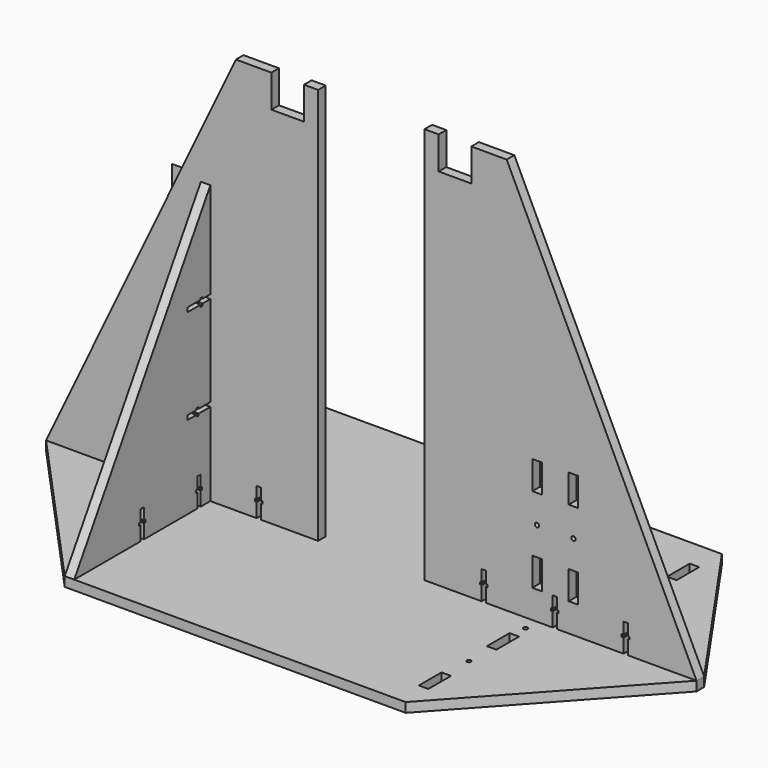
from build123d import *

# Parameters (mm, degrees)
F0_W     = 6.7
F0_H     = 20
F0_R     = 1.5
F1_DEPTH = 6.7
F3_DEPTH = 6.7
F4_R     = 1.5
F5_DEPTH = 25
F7_DEPTH = 6.7
F8_W     = 6.7
F8_H     = 20
F8_R     = 1.5
F8_W_2   = 20
F8_H_2   = 6.7
F9_DEPTH = 6.7


with BuildPart() as f1:
    # F0 (on Front) → F1 (new body)
    with BuildSketch(Plane.XZ):
        Polygon((-55.1449356675, 306.105045557), (-65.1449356675, 306.105045557), (-65.1449356675, 283.105045557), (-88.1449356675, 283.105045557), (-88.1449356675, 306.105045557), (-113.1449356675, 306.105045557), (-247.0069974661, 26.105045557), (-222.0069974661, 26.105045557), (-222.0069974661, 19.405045557), (-202.0069974661, 19.405045557), (-202.0069974661, 26.105045557), (-198.5069974661, 26.105045557), (-198.5069974661, 36.105045557), (-199.7569974661, 36.105045557), (-199.7569974661, 37.905045557), (-198.5069974661, 37.905045557), (-198.5069974661, 46.105045557), (-195.5069974661, 46.105045557), (-195.5069974661, 37.905045557), (-194.2569974661, 37.905045557), (-194.2569974661, 36.105045557), (-195.5069974661, 36.105045557), (-195.5069974661, 26.105045557), (-192.0069974661, 26.105045557), (-192.0069974661, 19.405045557), (-172.0069974661, 19.405045557), (-172.0069974661, 26.105045557), (-148.5069974661, 26.105045557), (-148.5069974661, 36.105045557), (-149.7569974661, 36.105045557), (-149.7569974661, 37.905045557), (-148.5069974661, 37.905045557), (-148.5069974661, 46.105045557), (-145.5069974661, 46.105045557), (-145.5069974661, 37.905045557), (-144.2569974661, 37.905045557), (-144.2569974661, 36.105045557), (-145.5069974661, 36.105045557), (-145.5069974661, 26.105045557), (-122.0069974661, 26.105045557), (-122.0069974661, 19.405045557), (-102.0069974661, 19.405045557), (-102.0069974661, 26.105045557), (-98.5069974661, 26.105045557), (-98.5069974661, 36.105045557), (-99.7569974661, 36.105045557), (-99.7569974661, 37.905045557), (-98.5069974661, 37.905045557), (-98.5069974661, 46.105045557), (-95.5069974661, 46.105045557), (-95.5069974661, 37.905045557), (-94.2569974661, 37.905045557), (-94.2569974661, 36.105045557), (-95.5069974661, 36.105045557), (-95.5069974661, 26.105045557), (-92.0069974661, 26.105045557), (-92.0069974661, 19.405045557), (-72.0069974661, 19.405045557), (-72.0069974661, 26.105045557), (-55.1449356675, 26.105045557), align=None)
        with Locations((-160.2069974661, 56.105045557)):
            Rectangle(F0_W, F0_H, mode=Mode.SUBTRACT)
        with Locations((-134.5069974661, 56.105045557)):
            Rectangle(F0_W, F0_H, mode=Mode.SUBTRACT)
        with Locations((-160.2069974661, 86.105045557)):
            Circle(F0_R, mode=Mode.SUBTRACT)
        with Locations((-134.5069974661, 86.105045557)):
            Circle(F0_R, mode=Mode.SUBTRACT)
        with Locations((-160.2069974661, 116.105045557)):
            Rectangle(F0_W, F0_H, mode=Mode.SUBTRACT)
        with Locations((-134.5069974661, 116.105045557)):
            Rectangle(F0_W, F0_H, mode=Mode.SUBTRACT)
    extrude(amount=F1_DEPTH)

    # F4 (on face) → F5 (cut)
    with BuildSketch(Plane(origin=(0, 0, 0), x_dir=(-1, 0, 0), z_dir=(0, 1, 0))):
        with Locations((134.5069974661, 153.039291501)):
            Circle(F4_R)
        with Locations((160.2069974661, 153.039291501)):
            Circle(F4_R)
        with Locations((-99.2171261311, 153.039291501)):
            Circle(F4_R)
        with Locations((-124.9171261311, 153.039291501)):
            Circle(F4_R)
    extrude(amount=-F5_DEPTH, mode=Mode.SUBTRACT)


with BuildPart() as f1b:
    # F0 (on Front) → F1, piece 2 (new body)
    with BuildSketch(Plane.XZ):
        Polygon((158.9671261311, 36.105045557), (158.9671261311, 37.905045557), (160.2171261311, 37.905045557), (160.2171261311, 46.105045557), (163.2171261311, 46.105045557), (163.2171261311, 37.905045557), (164.4671261311, 37.905045557), (164.4671261311, 36.105045557), (163.2171261311, 36.105045557), (163.2171261311, 26.105045557), (166.7171261311, 26.105045557), (166.7171261311, 19.405045557), (186.7171261311, 19.405045557), (186.7171261311, 26.105045557), (211.7171261311, 26.105045557), (77.8550643325, 306.105045557), (52.8550643325, 306.105045557), (52.8550643325, 283.105045557), (29.8550643325, 283.105045557), (29.8550643325, 306.105045557), (19.8550643325, 306.105045557), (19.8550643325, 26.105045557), (36.7171261311, 26.105045557), (36.7171261311, 19.405045557), (56.7171261311, 19.405045557), (56.7171261311, 26.105045557), (60.2171261311, 26.105045557), (60.2171261311, 36.105045557), (58.9671261311, 36.105045557), (58.9671261311, 37.905045557), (60.2171261311, 37.905045557), (60.2171261311, 46.105045557), (63.2171261311, 46.105045557), (63.2171261311, 37.905045557), (64.4671261311, 37.905045557), (64.4671261311, 36.105045557), (63.2171261311, 36.105045557), (63.2171261311, 26.105045557), (66.7171261311, 26.105045557), (66.7171261311, 19.405045557), (86.7171261311, 19.405045557), (86.7171261311, 26.105045557), (110.2171261311, 26.105045557), (110.2171261311, 36.105045557), (108.9671261311, 36.105045557), (108.9671261311, 37.905045557), (110.2171261311, 37.905045557), (110.2171261311, 46.105045557), (113.2171261311, 46.105045557), (113.2171261311, 37.905045557), (114.4671261311, 37.905045557), (114.4671261311, 36.105045557), (113.2171261311, 36.105045557), (113.2171261311, 26.105045557), (136.7171261311, 26.105045557), (136.7171261311, 19.405045557), (156.7171261311, 19.405045557), (156.7171261311, 26.105045557), (160.2171261311, 26.105045557), (160.2171261311, 36.105045557), align=None)
        with Locations((99.2171261311, 56.105045557)):
            Rectangle(F0_W, F0_H, mode=Mode.SUBTRACT)
        with Locations((124.9171261311, 56.105045557)):
            Rectangle(F0_W, F0_H, mode=Mode.SUBTRACT)
        with Locations((99.2171261311, 86.105045557)):
            Circle(F0_R, mode=Mode.SUBTRACT)
        with Locations((124.9171261311, 86.105045557)):
            Circle(F0_R, mode=Mode.SUBTRACT)
        with Locations((99.2171261311, 116.105045557)):
            Rectangle(F0_W, F0_H, mode=Mode.SUBTRACT)
        with Locations((124.9171261311, 116.105045557)):
            Rectangle(F0_W, F0_H, mode=Mode.SUBTRACT)
    extrude(amount=F1_DEPTH)


with BuildPart() as f3:
    # F2 (on face) → F3 (new body)
    with BuildSketch(Plane(origin=(-131.1569974661, 0, 0), x_dir=(0, -1, 0), z_dir=(-1, 0, 0))):
        Polygon((6.7, 126.105045557), (0, 126.105045557), (0, 106.105045557), (6.7, 106.105045557), (6.7, 87.605045557), (17.0851126313, 87.605045557), (17.0851126313, 88.855045557), (18.8851126313, 88.855045557), (18.8851126313, 87.605045557), (26.7, 87.605045557), (26.7, 84.605045557), (18.8851126313, 84.605045557), (18.8851126313, 83.355045557), (17.0851126313, 83.355045557), (17.0851126313, 84.605045557), (6.7, 84.605045557), (6.7, 66.105045557), (0, 66.105045557), (0, 46.105045557), (6.7, 46.105045557), (6.7, 26.105045557), (15.2, 26.105045557), (15.2, 36.105045557), (13.95, 36.105045557), (13.95, 37.905045557), (15.2, 37.905045557), (15.2, 46.105045557), (18.2, 46.105045557), (18.2, 37.905045557), (19.45, 37.905045557), (19.45, 36.105045557), (18.2, 36.105045557), (18.2, 26.105045557), (26.7, 26.105045557), (26.7, 19.405045557), (46.7, 19.405045557), (46.7, 26.105045557), (65.2, 26.105045557), (65.2, 36.105045557), (63.95, 36.105045557), (63.95, 37.905045557), (65.2, 37.905045557), (65.2, 46.105045557), (68.2, 46.105045557), (68.2, 37.905045557), (69.45, 37.905045557), (69.45, 36.105045557), (68.2, 36.105045557), (68.2, 26.105045557), (86.7, 26.105045557), (86.7, 19.405045557), (106.7, 19.405045557), (106.7, 26.105045557), (126.7, 26.105045557), (6.7, 222.1991419792), (6.7, 154.539291501), (13.4459044784, 154.539291501), (13.4459044784, 155.6246094704), (15.2459044784, 155.6246094704), (15.2459044784, 154.539291501), (26.7, 154.539291501), (26.7, 151.539291501), (15.2459044784, 151.539291501), (15.2459044784, 150.1246094704), (13.4459044784, 150.1246094704), (13.4459044784, 151.539291501), (6.7, 151.539291501), align=None)
    extrude(amount=F3_DEPTH)


with BuildPart() as f7:
    # F6 (on face) → F7 (new body)
    with BuildSketch(Plane(origin=(-156.8569974661, 0, 0), x_dir=(0, -1, 0), z_dir=(-1, 0, 0))):
        Polygon((6.7, 106.105045557), (6.7, 126.105045557), (0, 126.105045557), (0, 151.539291501), (-6.7459044784, 151.539291501), (-6.7459044784, 150.1246094704), (-8.5459044784, 150.1246094704), (-8.5459044784, 151.539291501), (-20, 151.539291501), (-20, 154.539291501), (-8.5459044784, 154.539291501), (-8.5459044784, 155.6246094704), (-6.7459044784, 155.6246094704), (-6.7459044784, 154.539291501), (0, 154.539291501), (0, 222.1991419792), (-120, 26.105045557), (-100, 26.105045557), (-100, 19.405045557), (-80, 19.405045557), (-80, 26.105045557), (-61.5, 26.105045557), (-61.5, 36.105045557), (-62.75, 36.105045557), (-62.75, 37.905045557), (-61.5, 37.905045557), (-61.5, 46.105045557), (-58.5, 46.105045557), (-58.5, 37.905045557), (-57.25, 37.905045557), (-57.25, 36.105045557), (-58.5, 36.105045557), (-58.5, 26.105045557), (-40, 26.105045557), (-40, 19.405045557), (-20, 19.405045557), (-20, 26.105045557), (-11.5, 26.105045557), (-11.5, 36.105045557), (-12.75, 36.105045557), (-12.75, 37.905045557), (-11.5, 37.905045557), (-11.5, 46.105045557), (-8.5, 46.105045557), (-8.5, 37.905045557), (-7.25, 37.905045557), (-7.25, 36.105045557), (-8.5, 36.105045557), (-8.5, 26.105045557), (0, 26.105045557), (0, 46.105045557), (6.7, 46.105045557), (6.7, 66.105045557), (0, 66.105045557), (0, 84.605045557), (-10.3851126313, 84.605045557), (-10.3851126313, 83.355045557), (-12.1851126313, 83.355045557), (-12.1851126313, 84.605045557), (-20, 84.605045557), (-20, 87.605045557), (-12.1851126313, 87.605045557), (-12.1851126313, 88.855045557), (-10.3851126313, 88.855045557), (-10.3851126313, 87.605045557), (0, 87.605045557), (0, 106.105045557), align=None)
    extrude(amount=F7_DEPTH)


with BuildPart() as f9:
    # F8 (on face) → F9 (new body)
    with BuildSketch(Plane(origin=(0, 0, 26.105045557), x_dir=(1, 0, 0), z_dir=(0, 0, -1))):
        Polygon((-137.8569974661, 126.7), (-247.0069974661, 6.7), (-247.0069974661, 0), (-163.5569974661, -120), (-156.8569974661, -120), (-17.6449356675, -120), (121.5671261311, -120), (128.2671261311, -120), (211.7171261311, 0), (211.7171261311, 6.7), (102.5671261311, 126.7), (95.8671261311, 126.7), (-17.6449356675, 126.7), (-131.1569974661, 126.7), align=None)
        with Locations((-160.2069974661, -90)):
            Rectangle(F8_W, F8_H, mode=Mode.SUBTRACT)
        with Locations((-160.2069974661, -60)):
            Circle(F8_R, mode=Mode.SUBTRACT)
        with Locations((-160.2069974661, -30)):
            Rectangle(F8_W, F8_H, mode=Mode.SUBTRACT)
        with Locations((-160.2069974661, -10)):
            Circle(F8_R, mode=Mode.SUBTRACT)
        with Locations((124.9171261311, -90)):
            Rectangle(F8_W, F8_H, mode=Mode.SUBTRACT)
        with Locations((124.9171261311, -60)):
            Circle(F8_R, mode=Mode.SUBTRACT)
        with Locations((124.9171261311, -30)):
            Rectangle(F8_W, F8_H, mode=Mode.SUBTRACT)
        with Locations((124.9171261311, -10)):
            Circle(F8_R, mode=Mode.SUBTRACT)
        with Locations((-212.0069974661, 3.35)):
            Rectangle(F8_W_2, F8_H_2, mode=Mode.SUBTRACT)
        with Locations((-197.0069974661, 3.35)):
            Circle(F8_R, mode=Mode.SUBTRACT)
        with Locations((-182.0069974661, 3.35)):
            Rectangle(F8_W_2, F8_H_2, mode=Mode.SUBTRACT)
        with Locations((-147.0069974661, 3.35)):
            Circle(F8_R, mode=Mode.SUBTRACT)
        with Locations((-134.5069974661, 16.7)):
            Circle(F8_R, mode=Mode.SUBTRACT)
        with Locations((-134.5069974661, 36.7)):
            Rectangle(F8_W, F8_H, mode=Mode.SUBTRACT)
        with Locations((-112.0069974661, 3.35)):
            Rectangle(F8_W_2, F8_H_2, mode=Mode.SUBTRACT)
        with Locations((-82.0069974661, 3.35)):
            Rectangle(F8_W_2, F8_H_2, mode=Mode.SUBTRACT)
        with Locations((-134.5069974661, 66.7)):
            Circle(F8_R, mode=Mode.SUBTRACT)
        with Locations((-134.5069974661, 96.7)):
            Rectangle(F8_W, F8_H, mode=Mode.SUBTRACT)
        with Locations((46.7171261311, 3.35)):
            Rectangle(F8_W_2, F8_H_2, mode=Mode.SUBTRACT)
        with Locations((76.7171261311, 3.35)):
            Rectangle(F8_W_2, F8_H_2, mode=Mode.SUBTRACT)
        with Locations((111.7171261311, 3.35)):
            Circle(F8_R, mode=Mode.SUBTRACT)
        with Locations((99.2171261311, 16.7)):
            Circle(F8_R, mode=Mode.SUBTRACT)
        with Locations((146.7171261311, 3.35)):
            Rectangle(F8_W_2, F8_H_2, mode=Mode.SUBTRACT)
        with Locations((161.7171261311, 3.35)):
            Circle(F8_R, mode=Mode.SUBTRACT)
        with Locations((176.7171261311, 3.35)):
            Rectangle(F8_W_2, F8_H_2, mode=Mode.SUBTRACT)
        with Locations((99.2171261311, 36.7)):
            Rectangle(F8_W, F8_H, mode=Mode.SUBTRACT)
        with Locations((99.2171261311, 66.7)):
            Circle(F8_R, mode=Mode.SUBTRACT)
        with Locations((99.2171261311, 96.7)):
            Rectangle(F8_W, F8_H, mode=Mode.SUBTRACT)
    extrude(amount=F9_DEPTH)


solid = Compound([f1.part, f1b.part, f3.part, f7.part, f9.part])
